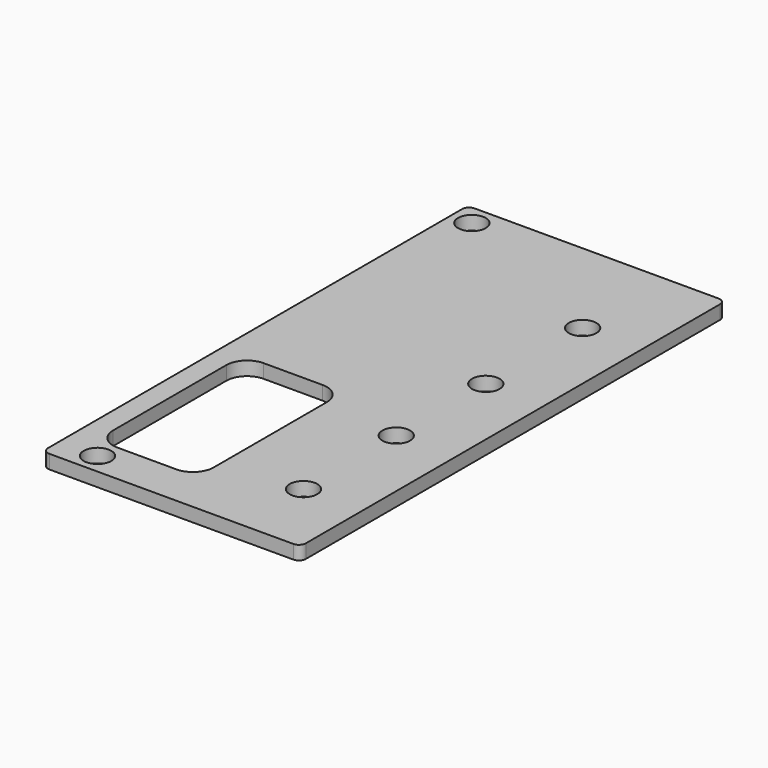
from build123d import *

# Parameters (mm, degrees)
F0_W     = 37.35
F0_H     = 77
F0_R     = 2
F0_W_2   = 14.55
F0_H_2   = 26.48
F1_DEPTH = 2
F2_R     = 3
F3_R     = 1


# Not quite as in the source:
# - a feature of the source that left no trace in its solid (it failed there, or was rolled back) is left out


with BuildPart() as f1:
    # F0 (on Top) → F1 (new body)
    with BuildSketch(Plane.XY):
        Rectangle(F0_W, F0_H)
        with Locations((-13.105, -35.5)):
            Circle(F0_R, mode=Mode.SUBTRACT)
        with Locations((-8.35, -19.26)):
            Rectangle(F0_W_2, F0_H_2, mode=Mode.SUBTRACT)
        with Locations((10.175, -27.3)):
            Circle(F0_R, mode=Mode.SUBTRACT)
        with Locations((10.175, -10.5)):
            Circle(F0_R, mode=Mode.SUBTRACT)
        with Locations((-15.675, 35.5)):
            Circle(F0_R, mode=Mode.SUBTRACT)
        with Locations((10.175, 5.72)):
            Circle(F0_R, mode=Mode.SUBTRACT)
        with Locations((10.175, 23.25)):
            Circle(F0_R, mode=Mode.SUBTRACT)
    extrude(amount=F1_DEPTH)

    # F2
    f2_edges = [f1.edges().sort_by_distance(p)[0] for p in [
        (-1.075, -6.02, 1),
        (-1.075, -32.5, 1),
        (-15.625, -32.5, 1),
        (-15.625, -6.02, 1),
    ]]
    fillet(f2_edges, radius=F2_R)

    # F3
    f3_edges = [f1.edges().sort_by_distance(p)[0] for p in [
        (-18.675, -38.5, 1),
        (18.675, -38.5, 1),
        (18.675, 38.5, 1),
        (-18.675, 38.5, 1),
    ]]
    fillet(f3_edges, radius=F3_R)


solid = f1.part
